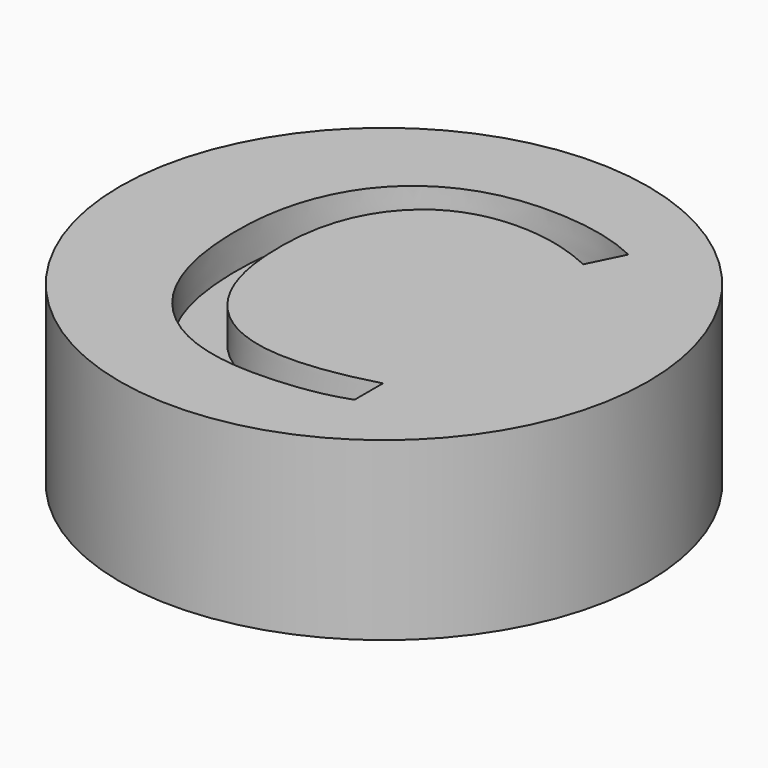
from build123d import *

# Parameters (mm, degrees)
F0_R         = 19.05
F1_DEPTH     = 12.7
F3_START     = 10.16
F2_TEXT_SIZE = 35.2777777778
F3_DEPTH     = 2.54


# Not quite as in the source:
# - Text() gives the source's letters only with a copy of the font that has no kerning and outlines rounded to 1/6400 em; it was checked with that copy


with BuildPart() as f1:
    # F0 (on Top) → F1 (new body)
    with BuildSketch(Plane.XY):
        Circle(F0_R)
    extrude(amount=F1_DEPTH)

    # F2 (on Top) → F3 (cut)
    with BuildSketch(Plane.XY.offset(F3_START)):
        with Locations((-12.7, -12.7)):
            Text('C', F2_TEXT_SIZE, font='Open Sans', text_align=(TextAlign.LEFT, TextAlign.BOTTOM))
    extrude(amount=F3_DEPTH, mode=Mode.SUBTRACT)


solid = f1.part
